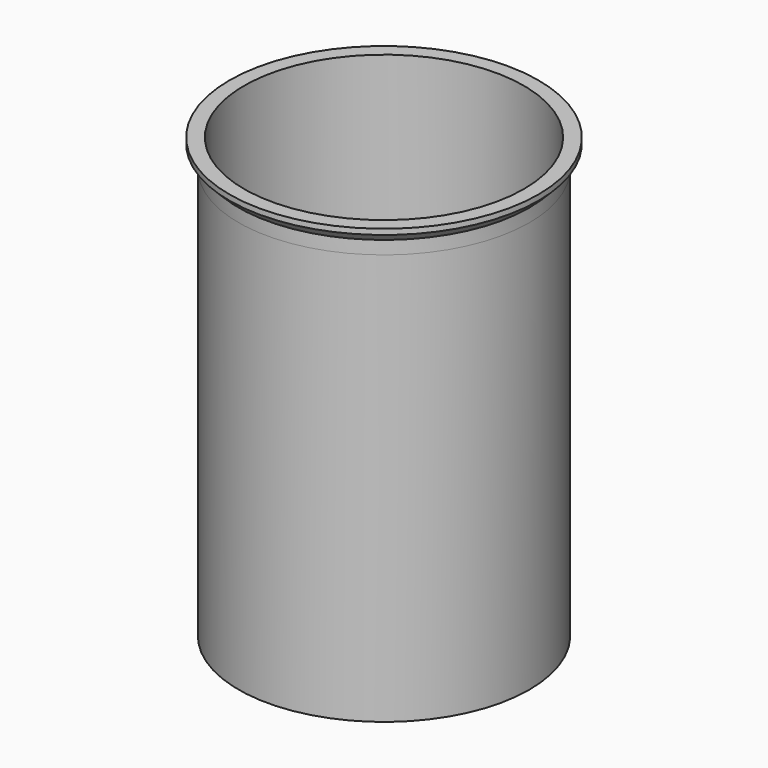
from build123d import *

# Parameters (mm, degrees)
F0_R        = 33.655
F0_R_2      = 32.385
F1_DEPTH    = 101.6
F2_R        = 33.3089939783
F3_DEPTH    = 2.54
F4_R        = 32.385
F4_R_2      = 3.175
F5_DEPTH    = 25.4
F6_R        = 35.7704476133
F6_R_2      = 33.0207785817
F7_DEPTH    = 6.35
F8_S5_R     = 33.655
F8_T6_DEPTH = 85


# Not quite as in the source:
# - a fillet or chamfer that OpenCascade refuses, or shapes differently, is made with other operations: its cross-section is extruded or revolved along the edge and cut away or added


with BuildPart() as f1:
    # F0 (on Top) → F1 (new body)
    with BuildSketch(Plane.XY):
        Circle(F0_R)
        Circle(F0_R_2, mode=Mode.SUBTRACT)
    extrude(amount=F1_DEPTH)

    # F2 (on Top) → F3 (join)
    with BuildSketch(Plane.XY):
        Circle(F2_R)
    extrude(amount=F3_DEPTH)

    # F4 (on face) → F5 (cut)
    with BuildSketch(Plane(origin=(0, 0, 0), x_dir=(1, 0, 0), z_dir=(0, 0, -1))):
        Circle(F4_R)
        with Locations((-7.9374271012, -25.5353750872)):
            Circle(F4_R_2, mode=Mode.SUBTRACT)
        with Locations((-21.4308303044, -15.993049812)):
            Circle(F4_R_2, mode=Mode.SUBTRACT)
        with Locations((-26.7383847386, -0.3419230925)):
            Circle(F4_R_2, mode=Mode.SUBTRACT)
        with Locations((-3.6135736787, -11.1214362212)):
            Circle(F4_R_2, mode=Mode.SUBTRACT)
        with Locations((8.5878034715, -25.3240549945)):
            Circle(F4_R_2, mode=Mode.SUBTRACT)
        with Locations((9.4604587116, -6.8734255884)):
            Circle(F4_R_2, mode=Mode.SUBTRACT)
        with Locations((21.8327850068, -15.4398066269)):
            Circle(F4_R_2, mode=Mode.SUBTRACT)
        with Locations((-21.8327850068, 15.4398066269)):
            Circle(F4_R_2, mode=Mode.SUBTRACT)
        with Locations((-11.6937700659, 0)):
            Circle(F4_R_2, mode=Mode.SUBTRACT)
        with Locations((-3.6135736787, 11.1214362212)):
            Circle(F4_R_2, mode=Mode.SUBTRACT)
        with Locations((-8.5878034715, 25.3240549945)):
            Circle(F4_R_2, mode=Mode.SUBTRACT)
        Circle(F4_R_2, mode=Mode.SUBTRACT)
        with Locations((9.4604587116, 6.8734255884)):
            Circle(F4_R_2, mode=Mode.SUBTRACT)
        with Locations((26.7383847386, 0.3419230925)):
            Circle(F4_R_2, mode=Mode.SUBTRACT)
        with Locations((21.4308303044, 15.993049812)):
            Circle(F4_R_2, mode=Mode.SUBTRACT)
        with Locations((7.9374271012, 25.5353750872)):
            Circle(F4_R_2, mode=Mode.SUBTRACT)
    extrude(amount=-F5_DEPTH, mode=Mode.SUBTRACT)

    # F6 (on face) → F7 (join)
    with BuildSketch(Plane.XY.offset(101.6)):
        Circle(F6_R)
        Circle(F6_R_2, mode=Mode.SUBTRACT)
    extrude(amount=-F7_DEPTH)

    # F8: chamfer of 5.08 on 1 edges, made by hand


with BuildPart() as f8_tool2:
    # F8_s3 → F8_t4 (revolve)
    with BuildSketch(Plane.XZ):
        with BuildLine():
            Line((30.5467635153, 95.1063159021), (35.9141317112, 100.4736840979))
            Line((35.9141317112, 100.4736840979), (36.0157317112, 100.4736840979))
            ThreePointArc((36.0157317112, 100.4736840979), (35.8720476133, 97.861842049), (35.8720476133, 95.25))
            Line((35.8720476133, 95.25), (35.7704476133, 95.1484))
            ThreePointArc((35.7704476133, 95.1484), (33.1586055643, 95.1484), (30.5467635153, 95.0047159021))
            Line((30.5467635153, 95.0047159021), (30.5467635153, 95.1063159021))
        make_face()
    revolve(axis=Axis((0, 0, 95.25), (0, 0, 1)))

    # F8_s5 → F8_t6 (cut, symmetric)
    with BuildSketch(Plane.XY.offset(96.6)):
        Circle(F8_S5_R)
    extrude(amount=F8_T6_DEPTH, both=True, mode=Mode.SUBTRACT)


with BuildPart() as f1_1:
    add(f1.part)

    # F8_t1: cut F8_tool2
    add(f8_tool2.part, mode=Mode.SUBTRACT)


solid = f1_1.part
